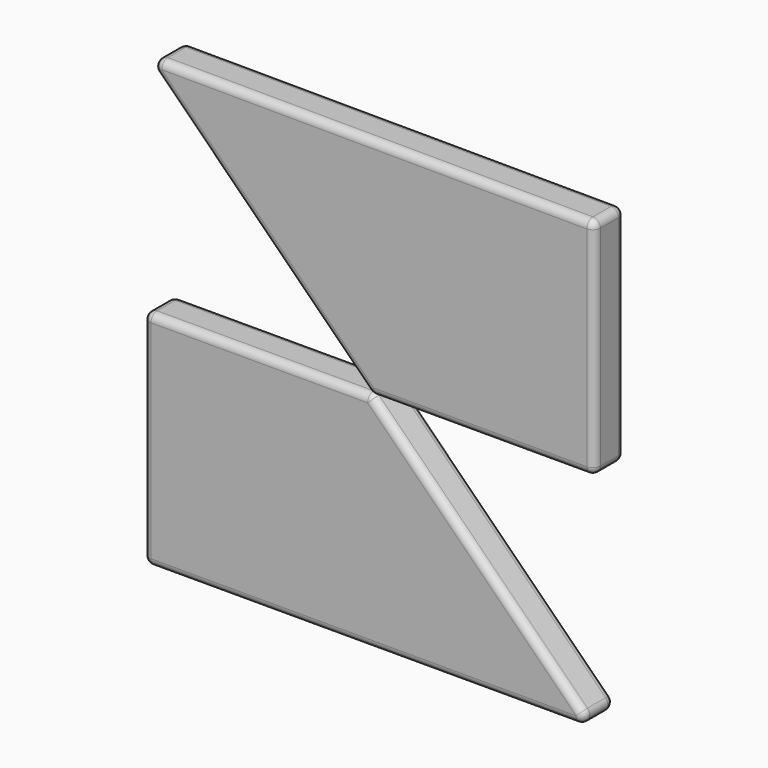
from build123d import *

# Parameters (mm, degrees)
F1_DEPTH = 12.7
F2_R     = 2.54
F2_2_R   = 2.54
F3_R     = 2.54
F3_2_R   = 2.54


with BuildPart() as f1:
    # F0 (on Front) → F1 (new body)
    with BuildSketch(Plane.XZ):
        Polygon((75.2567246384, -74.9815637702), (0, 0), (-76.5130594373, -74.9815637702), align=None)
        Polygon((-76.5130594373, -74.9815637702), (0, 0), (-76.5130594373, 0), align=None)
    extrude(amount=F1_DEPTH)

    # F2
    f2_edges = [f1.edges().sort_by_distance(p)[0] for p in [
        (0, -6.35, 0),
    ]]
    fillet(f2_edges, radius=F2_R)

    # F3
    f3_edges = [f1.edges().sort_by_distance(p)[0] for p in [
        (-76.513059, -6.35, 0),
        (-76.513059, -6.35, -74.981564),
        (-76.513059, 0, -37.490782),
        (-76.513059, -12.7, -37.490782),
        (-38.781219, 0, 0),
        (-1.049378, -6.35, 0),
        (-38.781219, -12.7, 0),
        (75.256725, -6.35, -74.981564),
        (-0.628167, 0, -74.981564),
        (-0.628167, -12.7, -74.981564),
        (38.000052, 0, -37.861113),
        (0.74338, -6.35, -0.740662),
        (38.000052, -12.7, -37.861113),
        (-0.079512, 0, -0.192457),
        (-0.079512, -12.7, -0.192457),
    ]]
    fillet(f3_edges, radius=F3_R)


with BuildPart() as f1b:
    # F0 (on Front) → F1, piece 2 (new body)
    with BuildSketch(Plane.XZ):
        Polygon((75.2567246384, 75.5328952683), (0, 0), (75.2567246384, 0), align=None)
        Polygon((75.2567246384, 75.5328952683), (-76.5130594373, 76.233305037), (0, 0), align=None)
    extrude(amount=F1_DEPTH)

    # F2#2
    f2_2_edges = [f1b.edges().sort_by_distance(p)[0] for p in [
        (-76.513059, -6.35, 76.233305),
        (-38.25653, 0, 38.116653),
        (-38.25653, -12.7, 38.116653),
        (75.256725, -6.35, 75.532895),
        (-0.628167, 0, 75.8831),
        (-0.628167, -12.7, 75.8831),
        (75.256725, -6.35, 0),
        (75.256725, 0, 37.766448),
        (75.256725, -12.7, 37.766448),
        (37.628362, 0, 0),
        (37.628362, -12.7, 0),
    ]]
    fillet(f2_2_edges, radius=F2_2_R)

    # F3#2
    f3_2_edges = [f1b.edges().sort_by_distance(p)[0] for p in [
        (0, -6.35, 0),
    ]]
    fillet(f3_2_edges, radius=F3_2_R)


solid = Compound([f1.part, f1b.part])
